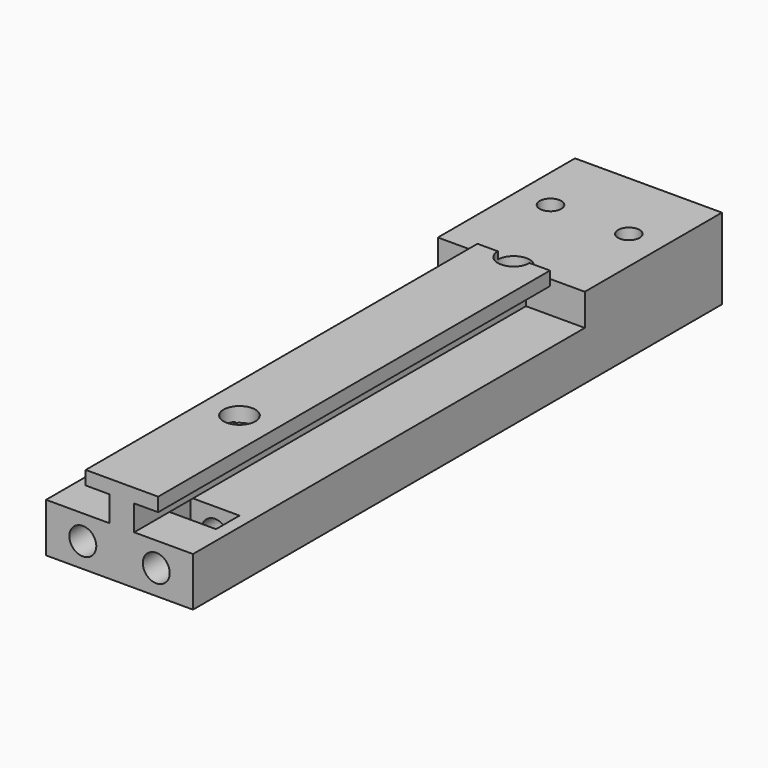
from build123d import *

# Parameters (mm, degrees)
F0_R            = 2.5000000706
F0_R_2          = 2.5000000298
F0_W            = 4.9999998882
F0_H            = 5.2
F1_DEPTH        = 100
F3_DEPTH        = 35
F6_D            = 4.4
F6_DEPTH        = 40
F6_TIP          = 1.3218933619
F5_W            = 10
F5_H            = 6
F7_DEPTH        = 10
F9_D            = 5.5
F9_DEPTH        = 40
F9_TIP          = 1.6523667023
F11_D           = 3.3
F11_DEPTH       = 20
F11_START       = 1.4999997
F11_CBORE_D     = 6.5
F11_CBORE_DEPTH = 3
F11_TIP         = 0.9914200214
F12_DEPTH       = 4


# Not quite as in the source:
# - after a boolean that leaves OpenCascade's solid faulty, fix() repairs it
# - ends of sketch curves that miss each other by under 0.0002 mm in the source are joined
# - a feature names something its author has since deleted; it is built from what else it names


with BuildPart() as f1:
    # F0 (on Front) → F1 (new body)
    with BuildSketch(Plane.XZ):
        Polygon((-38.4980148883, 4.2457092745), (-38.4980148883, -5.7542903855), (-8.4980155588, -5.7542903855), (-8.4980155588, 4.2457092745), (-15.6109269008, 4.2457092745), (-20.5109269008, 4.2457092745), (-25.510926789, 4.2457092745), (-30.410926789, 4.2457092745), align=None)
        with Locations((-30.9980151824, -0.7542907016)):
            Circle(F0_R, mode=Mode.SUBTRACT)
        with Locations((-15.9980151584, -0.7062930843)):
            Circle(F0_R_2, mode=Mode.SUBTRACT)
        with Locations((-23.0109268449, 6.8457092745)):
            Rectangle(F0_W, F0_H)
        with Locations((-30.9980151824, -0.7542907016)):
            Circle(F0_R)
        with Locations((-15.9980151584, -0.7062930843)):
            Circle(F0_R_2)
        Polygon((-30.410926789, 12.2457092745), (-30.410926789, 9.4457092745), (-25.510926789, 9.4457092745), (-20.5109269008, 9.4457092745), (-15.6109269008, 9.4457092745), (-15.6109269008, 12.2457092745), align=None)
    extrude(amount=F1_DEPTH)

    # F2 (on face) → F3 (join)
    with BuildSketch(Plane(origin=(0, 0, 0), x_dir=(-1, 0, 0), z_dir=(0, 1, 0))):
        Polygon((8.4980155588, 10.7457096145), (8.4980155588, 4.2457092745), (20.5109269008, 4.2457092745), (20.5109269008, 9.4457092745), (15.6109269008, 9.4457092745), (15.6109269008, 10.7457096145), align=None)
        Polygon((25.510926789, 4.2457092745), (38.4980148883, 4.2457092745), (38.4980155588, 10.7457096145), (30.410926789, 10.7457096145), (30.410926789, 9.4457092745), (25.510926789, 9.4457092745), align=None)
        Polygon((8.4980155588, 4.2457092745), (8.4980155588, -5.7542903855), (38.4980155588, -5.7542903855), (38.4980155588, 4.2457092745), (25.510926789, 4.2457092745), (25.510926789, 9.4457092745), (30.410926789, 9.4457092745), (30.410926789, 10.7457096145), (15.6109269008, 10.7457096145), (15.6109269008, 9.4457092745), (20.5109269008, 9.4457092745), (20.5109269008, 4.2457092745), align=None)
    extrude(amount=F3_DEPTH)

    # F4: union 

    # F6
    with Locations(Plane(origin=(0, 0, -5.7542903855), x_dir=(1, 0, 0), z_dir=(0, 0, -1))):
        with Locations((-15.4980155588, -20), (-31.4980148883, -20)):
            Hole(F6_D / 2, depth=F6_DEPTH)
            with Locations((0, 0, -(F6_DEPTH + F6_TIP / 2))):  # 118° drill point
                Cone(0, F6_D / 2, F6_TIP, mode=Mode.SUBTRACT)

    # F5 (on face) → F7 (cut)
    with BuildSketch(Plane(origin=(0, 0, -5.7542903855), x_dir=(1, 0, 0), z_dir=(0, 0, -1))):
        with Locations((-15.9980155588, 88)):
            Rectangle(F5_W, F5_H)
        with Locations((-30.9980148883, 88)):
            Rectangle(F5_W, F5_H)
    extrude(amount=-F7_DEPTH, mode=Mode.SUBTRACT)

    add(f1.part.fix(), mode=Mode.REPLACE)

    # F9
    with Locations(Plane.XZ.offset(100)):
        with Locations((-30.9980151824, -0.7542907016), (-15.9980151584, -0.7062930843)):
            Hole(F9_D / 2, depth=F9_DEPTH)
            with Locations((0, 0, -(F9_DEPTH + F9_TIP / 2))):  # 118° drill point
                Cone(0, F9_D / 2, F9_TIP, mode=Mode.SUBTRACT)

    # F11
    # its depths count from where the whole tool has entered the part; down to there all is cleared
    with Locations(Plane.XY.offset(12.2457092745)):
        with Locations((-23.0109268449, 0, -F11_START), (-23.0109268449, -70, 0)):
            CounterBoreHole(F11_D / 2, F11_CBORE_D / 2, F11_CBORE_DEPTH, depth=F11_DEPTH)
            with Locations((0, 0, -(F11_DEPTH + F11_TIP / 2))):  # 118° drill point
                Cone(0, F11_D / 2, F11_TIP, mode=Mode.SUBTRACT)

    # F5 (on face) → F12 (cut)
    with BuildSketch(Plane(origin=(0, 0, -5.7542903855), x_dir=(1, 0, 0), z_dir=(0, 0, -1))):
        Polygon((-18.9980155588, -17.9792740578), (-18.9980155588, -22.0207259422), (-15.4980155588, -24.0414518843), (-11.9980155588, -22.0207259422), (-11.9980155588, -17.9792740578), (-15.4980155588, -15.9585481157), align=None)
        Polygon((-31.4247349717, -24.0407874712), (-27.9619503287, -21.9569314662), (-28.0352302453, -17.9161439951), (-31.5712948049, -15.9592125288), (-35.0340794479, -18.0430685338), (-34.9607995313, -22.0838560049), align=None)
    extrude(amount=-F12_DEPTH, mode=Mode.SUBTRACT)


solid = f1.part
